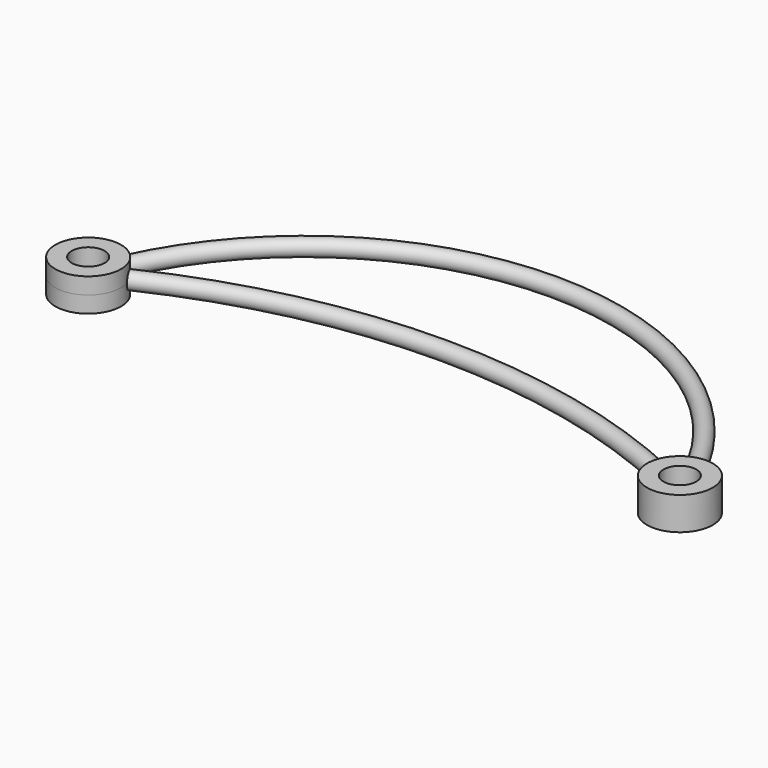
from build123d import *

# Parameters (mm, degrees)
F2_R     = 25.4
F2_R_2   = 21.742
F3_R     = 25.4
F3_R_2   = 21.742
F6_R     = 100
F6_R_2   = 50
F7_DEPTH = 50


with BuildPart() as f4:
    # F4: sweep along a path in F1
    with BuildLine(Plane.XY) as f4_path:
        ThreePointArc((810.7144863791, -440.4517624252), (0, -258.8062140954), (-810.7144863791, -440.4517624252))
    # F2 (on Right) → F4 (sweep)
    with BuildSketch(Plane.YZ):
        with Locations((-258.8062140954, 0)):
            Circle(F2_R)
        with Locations((-258.8062140954, 0)):
            Circle(F2_R_2, mode=Mode.SUBTRACT)
    sweep(path=f4_path.line)



with BuildPart() as f5:
    # F5: sweep along a path in F1
    with BuildLine(Plane.XY) as f5_path:
        ThreePointArc((863.0516210993, -392.5624434058), (0, 160.4350098154), (-863.0516210993, -392.5624434058))
    # F3 (on Right) → F5 (sweep)
    with BuildSketch(Plane.YZ):
        with Locations((160.4350098154, 0)):
            Circle(F3_R)
        with Locations((160.4350098154, 0)):
            Circle(F3_R_2, mode=Mode.SUBTRACT)
    sweep(path=f5_path.line)


with BuildPart() as f4_1:
    add(f4.part)

    add(f5.part)  # F7 merges F5
    # F6 (on Top) → F7 (join, symmetric)
    with BuildSketch(Plane.XY):
        with Locations((-900, -485.4861610273)):
            Circle(F6_R)
        with Locations((-900, -485.4861610273)):
            Circle(F6_R_2, mode=Mode.SUBTRACT)
        with Locations((900, -485.4861610273)):
            Circle(F6_R)
        with Locations((900, -485.4861610273)):
            Circle(F6_R_2, mode=Mode.SUBTRACT)
    extrude(amount=F7_DEPTH, both=True)


solid = f4_1.part
